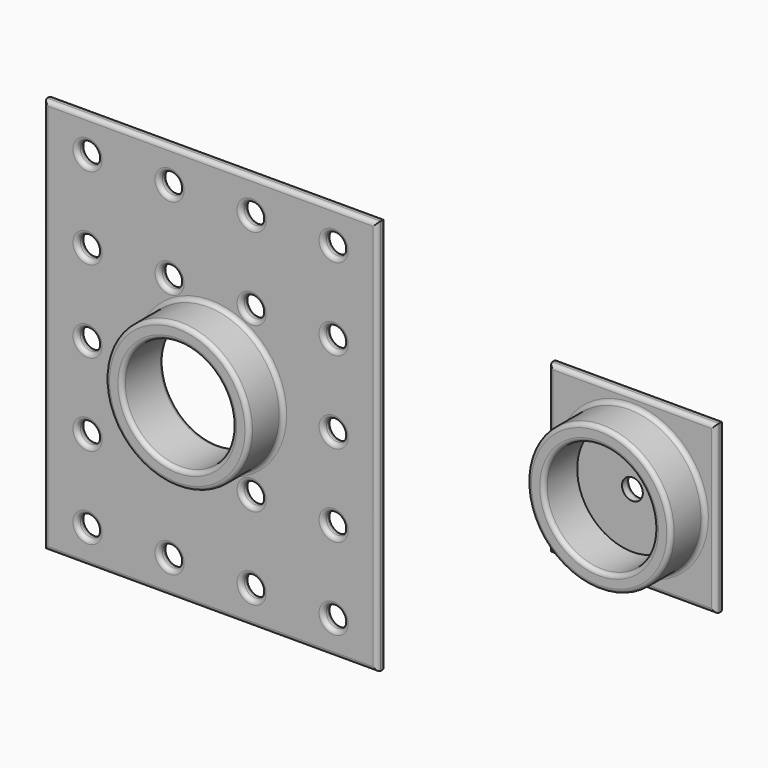
from build123d import *

# Parameters (mm, degrees)
F0_W     = 101.6
F0_H     = 120.65
F0_R     = 3.175
F0_R_2   = 21.9075
F0_R_3   = 16.8275
F1_DEPTH = 3.175
F2_DEPTH = 12.7
F3_R     = 1.27
F4_W     = 50.8
F4_H     = 50.8
F4_R     = 21.9075
F4_R_2   = 16.8275
F4_R_3   = 3.175
F5_DEPTH = 3.175
F6_DEPTH = 12.7
F7_R     = 1.27


with BuildPart() as f1:
    # F0 (on Front) → F1 (new body)
    with BuildSketch(Plane.XZ):
        Rectangle(F0_W, F0_H)
        with Locations((-37.5, -50)):
            Circle(F0_R, mode=Mode.SUBTRACT)
        with Locations((-12.5, -50)):
            Circle(F0_R, mode=Mode.SUBTRACT)
        with Locations((-37.5, -25)):
            Circle(F0_R, mode=Mode.SUBTRACT)
        with Locations((-12.5, -25)):
            Circle(F0_R, mode=Mode.SUBTRACT)
        with Locations((12.5, -50)):
            Circle(F0_R, mode=Mode.SUBTRACT)
        with Locations((37.5, -50)):
            Circle(F0_R, mode=Mode.SUBTRACT)
        with Locations((12.5, -25)):
            Circle(F0_R, mode=Mode.SUBTRACT)
        with Locations((37.5, -25)):
            Circle(F0_R, mode=Mode.SUBTRACT)
        with Locations((-37.5, 0)):
            Circle(F0_R, mode=Mode.SUBTRACT)
        with Locations((-37.5, 25)):
            Circle(F0_R, mode=Mode.SUBTRACT)
        Circle(F0_R_2, mode=Mode.SUBTRACT)
        with Locations((-12.5, 25)):
            Circle(F0_R, mode=Mode.SUBTRACT)
        with Locations((-37.5, 50)):
            Circle(F0_R, mode=Mode.SUBTRACT)
        with Locations((-12.5, 50)):
            Circle(F0_R, mode=Mode.SUBTRACT)
        with Locations((12.5, 25)):
            Circle(F0_R, mode=Mode.SUBTRACT)
        with Locations((37.5, 0)):
            Circle(F0_R, mode=Mode.SUBTRACT)
        with Locations((37.5, 25)):
            Circle(F0_R, mode=Mode.SUBTRACT)
        with Locations((12.5, 50)):
            Circle(F0_R, mode=Mode.SUBTRACT)
        with Locations((37.5, 50)):
            Circle(F0_R, mode=Mode.SUBTRACT)
        Circle(F0_R_2)
        Circle(F0_R_3, mode=Mode.SUBTRACT)
    extrude(amount=-F1_DEPTH)

    # F0 (on Front) → F2 (join)
    with BuildSketch(Plane.XZ):
        Circle(F0_R_2)
        Circle(F0_R_3, mode=Mode.SUBTRACT)
    extrude(amount=F2_DEPTH)

    # F3
    f3_edges = [f1.edges().sort_by_distance(p)[0] for p in [
        (-16.8275, -12.7, 0),
        (-21.9075, -12.7, 0),
        (-21.9075, 0, 0),
        (0, 0, 60.325),
        (50.8, 0, 0),
        (-50.8, 0, 0),
        (0, 0, -60.325),
        (-40.675, 0, -50),
        (-15.675, 0, -50),
        (-40.675, 0, -25),
        (-15.675, 0, -25),
        (9.325, 0, -50),
        (34.325, 0, -50),
        (9.325, 0, -25),
        (34.325, 0, -25),
        (-40.675, 0, 0),
        (-40.675, 0, 25),
        (-15.675, 0, 25),
        (-40.675, 0, 50),
        (-15.675, 0, 50),
        (9.325, 0, 25),
        (34.325, 0, 0),
        (34.325, 0, 25),
        (9.325, 0, 50),
        (34.325, 0, 50),
        (0, 3.175, 60.325),
        (-50.8, 3.175, 0),
        (0, 3.175, -60.325),
        (50.8, 3.175, 0),
        (-40.675, 3.175, -50),
        (-15.675, 3.175, -50),
        (-40.675, 3.175, -25),
        (-15.675, 3.175, -25),
        (9.325, 3.175, -50),
        (34.325, 3.175, -50),
        (9.325, 3.175, -25),
        (34.325, 3.175, -25),
        (-40.675, 3.175, 0),
        (-40.675, 3.175, 25),
        (-15.675, 3.175, 25),
        (-40.675, 3.175, 50),
        (-15.675, 3.175, 50),
        (9.325, 3.175, 25),
        (34.325, 3.175, 0),
        (34.325, 3.175, 25),
        (9.325, 3.175, 50),
        (34.325, 3.175, 50),
        (-16.8275, 3.175, 0),
    ]]
    fillet(f3_edges, radius=F3_R)


with BuildPart() as f5:
    # F4 (on Front) → F5 (new body, through all)
    with BuildSketch(Plane.XZ):
        with Locations((128.5328067183, 14.2264530718)):
            Rectangle(F4_W, F4_H)
        with Locations((128.5328067183, 14.2264530718)):
            Circle(F4_R, mode=Mode.SUBTRACT)
        with Locations((128.5328067183, 14.2264530718)):
            Circle(F4_R)
        with Locations((128.5328067183, 14.2264530718)):
            Circle(F4_R_2, mode=Mode.SUBTRACT)
        with Locations((128.5328067183, 14.2264530718)):
            Circle(F4_R_2)
        with Locations((128.5328067183, 14.2264530718)):
            Circle(F4_R_3, mode=Mode.SUBTRACT)
    extrude(amount=-F5_DEPTH)

    # F4 (on Front) → F6 (join, through all)
    with BuildSketch(Plane.XZ):
        with Locations((128.5328067183, 14.2264530718)):
            Circle(F4_R)
        with Locations((128.5328067183, 14.2264530718)):
            Circle(F4_R_2, mode=Mode.SUBTRACT)
    extrude(amount=F6_DEPTH)

    # F7
    f7_edges = [f5.edges().sort_by_distance(p)[0] for p in [
        (128.532807, 0, 39.626453),
        (153.932807, 0, 14.226453),
        (103.132807, 0, 14.226453),
        (128.532807, 0, -11.173547),
        (106.625307, 0, 14.226453),
        (128.532807, 3.175, 39.626453),
        (153.932807, 3.175, 14.226453),
        (103.132807, 3.175, 14.226453),
        (128.532807, 3.175, -11.173547),
        (125.357807, 3.175, 14.226453),
        (106.625307, -12.7, 14.226453),
        (111.705307, -12.7, 14.226453),
    ]]
    fillet(f7_edges, radius=F7_R)


solid = Compound([f1.part, f5.part])
